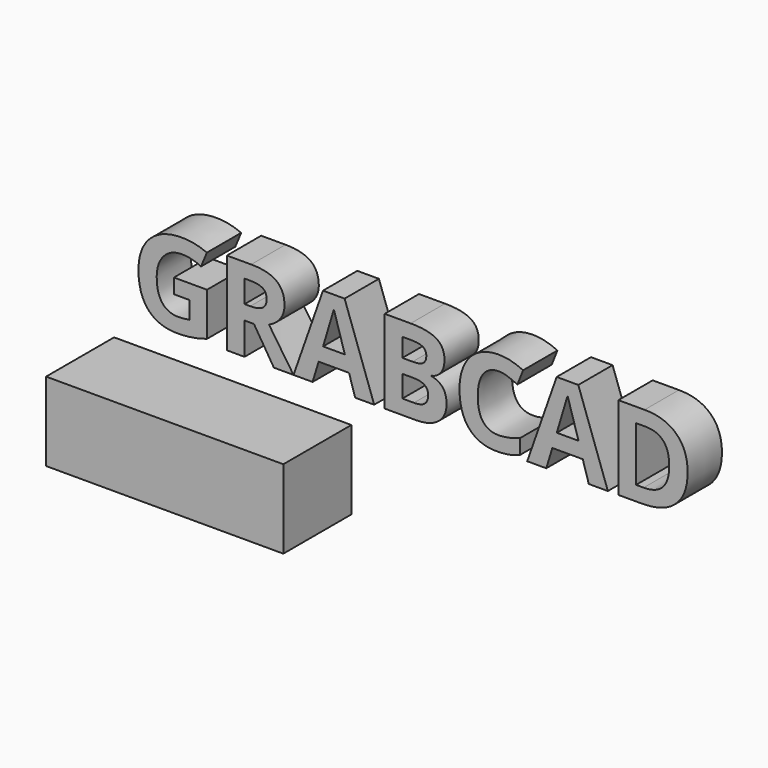
from build123d import *

# Parameters (mm, degrees)
F0_TEXT_SIZE = 33.2582302185
F1_DEPTH     = 12.2
F2_W         = 24.1885893047
F2_H         = 22.4028546363
F3_DEPTH     = 67.5


# Not quite as in the source:
# - Text() gives the source's letters only with a copy of the font that has no kerning and outlines rounded to 1/6400 em; it was checked with that copy


with BuildPart() as f1:
    # F0 (on Front) → F1 (new body)
    with BuildSketch(Plane.XZ):
        with Locations((-47.3856963217, 0)):
            Text('GRABCAD', F0_TEXT_SIZE, font='Open Sans', font_style=FontStyle.BOLD, text_align=(TextAlign.LEFT, TextAlign.BOTTOM))
    extrude(amount=F1_DEPTH)


with BuildPart() as f3:
    # F2 (on Right) → F3 (new body)
    with BuildSketch(Plane.YZ):
        with Locations((-5.4130870849, -30.9731913731)):
            Rectangle(F2_W, F2_H)
    extrude(amount=-F3_DEPTH)


solid = Compound([f1.part, f3.part])
